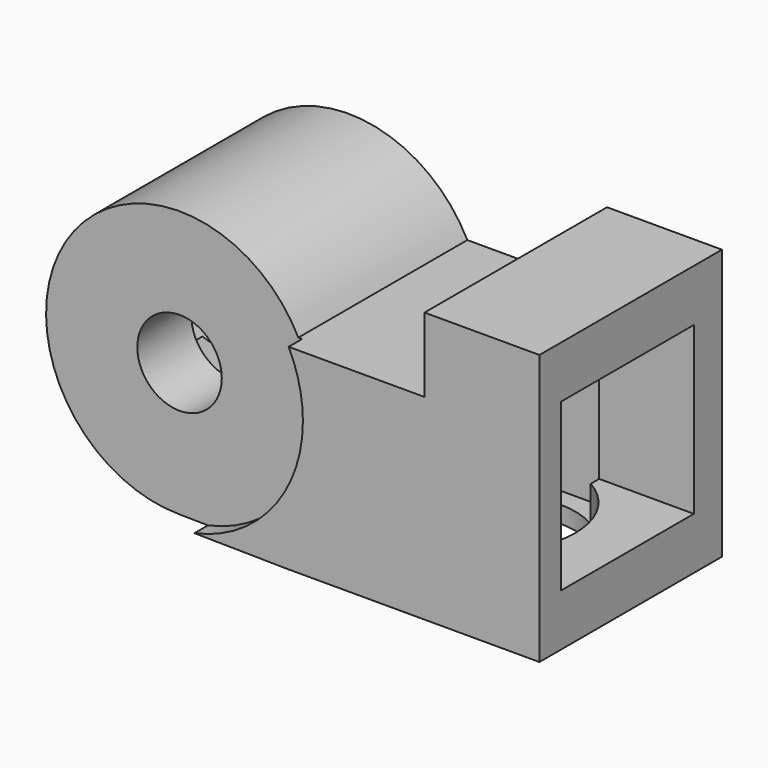
from build123d import *

# Parameters (mm, degrees)
F1_DEPTH  = 67.5
F3_W      = 49.2
F3_H      = 49.2
F4_DEPTH  = 28
F6_W      = 57.5
F6_H      = 48
F7_DEPTH  = 40
F9_DEPTH  = 5
F10_R     = 12.5
F11_DEPTH = 20
F13_R     = 34.5
F14_DEPTH = 37.5
F16_W     = 52.5
F16_H     = 48
F17_DEPTH = 25
F18_R     = 24.6
F19_DEPTH = 20


with BuildPart() as f1:
    # F0 (on Front) → F1 (new body)
    with BuildSketch(Plane.XZ):
        with BuildLine():
            ThreePointArc((-35.5098846553, 0.5000012368), (-7.5727771152, 12.0657876083), (4, 40))
            ThreePointArc((4, 40), (2.8997637092, 49.2578694674), (-0.3396530165, 58))
            ThreePointArc((-0.3396530165, 58), (-69.1964570083, 60.6106473718), (-35.5098846553, 0.5000012368))
        make_face()
        with BuildLine():
            ThreePointArc((-0.3396530165, 58), (2.8997637092, 49.2578694674), (4, 40))
            ThreePointArc((4, 40), (-7.5727771152, 12.0657876083), (-35.5098846553, 0.5000012368))
            Line((-35.5098846553, 0.5000012368), (0, 0))
            Line((0, 0), (75, 0))
            Line((75, 0), (75, 80))
            Line((75, 80), (41, 80))
            Line((41, 80), (41, 58))
            Line((41, 58), (-0.3396530165, 58))
        make_face()
    extrude(amount=-F1_DEPTH)

    # F3 (on offset) → F4 (cut)
    with BuildSketch(Plane.YZ.offset(75)):
        with Locations((32.5, 40)):
            Rectangle(F3_W, F3_H)
    extrude(amount=-F4_DEPTH, mode=Mode.SUBTRACT)

    # F6 (on offset) → F7 (cut)
    with BuildSketch(Plane.YZ.offset(47)):
        with Locations((33.75, 29)):
            Rectangle(F6_W, F6_H)
    extrude(amount=-F7_DEPTH, mode=Mode.SUBTRACT)

    # F8 (on face) → F9 (cut)
    with BuildSketch(Plane.XZ):
        with BuildLine():
            ThreePointArc((-27.0960278356, 0.3815289056), (-4.0308812273, 14.5059896511), (5, 40))
            ThreePointArc((5, 40), (3.9309299575, 49.2440122613), (0.7801598673, 58))
            Line((0.7801598673, 58), (-0.3396530165, 58))
            ThreePointArc((-0.3396530165, 58), (-69.1964570083, 60.6106473718), (-35.5098846553, 0.5000012368))
            Line((-35.5098846553, 0.5000012368), (-27.0960278356, 0.3815289056))
        make_face()
    extrude(amount=-F9_DEPTH, mode=Mode.SUBTRACT)

    # F10 (on face) → F11 (cut)
    with BuildSketch(Plane.XZ.offset(-5)):
        with Locations((-35.5, 40)):
            Circle(F10_R)
    extrude(amount=-F11_DEPTH, mode=Mode.SUBTRACT)

    # F13 (on offset) → F14 (cut)
    with BuildSketch(Plane.XZ.offset(-25)):
        with Locations((-35.5, 40)):
            Circle(F13_R)
    extrude(amount=-F14_DEPTH, mode=Mode.SUBTRACT)

    # F16 (on offset) → F17 (cut)
    with BuildSketch(Plane.YZ.offset(7)):
        with Locations((36.25, 29)):
            Rectangle(F16_W, F16_H)
    extrude(amount=-F17_DEPTH, mode=Mode.SUBTRACT)

    # F18 (on Top) → F19 (cut)
    with BuildSketch(Plane.XY):
        with Locations((-45, 32.5)):
            Circle(F18_R)
        with Locations((35, 32.5)):
            Circle(F18_R)
    extrude(amount=F19_DEPTH, mode=Mode.SUBTRACT)


solid = f1.part
